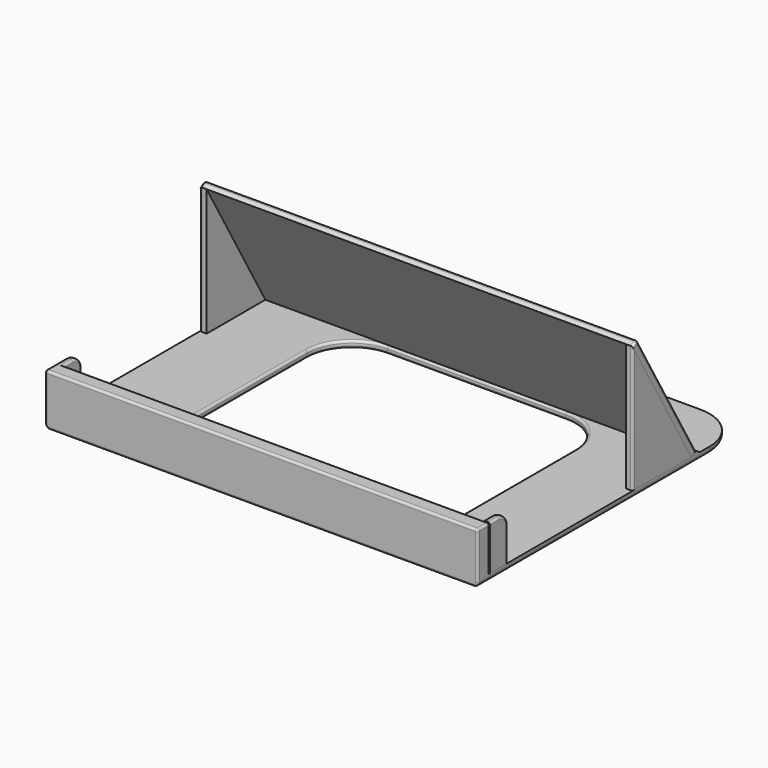
from build123d import *

# Parameters (mm, degrees)
F0_W          = 194
F0_H          = 150
F1_DEPTH      = 3
F2_W          = 6.9154556079
F2_H          = 20
F3_DEPTH      = 194
F5_DEPTH      = 3
F7_DEPTH      = 3
F8_W          = 194
F8_H          = 65.8179306876
F9_DEPTH      = 3
F11_DEPTH     = 194
F12_W         = 10
F12_H         = 20
F13_DEPTH     = 3
F14_R         = 5
F15_R         = 1
F16_R         = 1
F18_DEPTH     = 3
F19_R         = 1
F20_R         = 1
F21_R         = 1
F22_W         = 120
F22_H         = 112
F23_DEPTH     = 3.001
F24_R         = 20
F25_R         = 20
F26_R         = 2
F27_R         = 1
F28_R         = 1
F29_R         = 1
F30_T1_DEPTH  = 72
F30_T3_DEPTH  = 80
F30_T6_ANGLE  = 90
F30_T8_ANGLE  = 90
F30_T12_ANGLE = 111.4945483856
F30_T17_ANGLE = 111.4945483856
F31_R         = 1
F31_2_R       = 1


# Not quite as in the source:
# - a fillet or chamfer that OpenCascade refuses, or shapes differently, is made with other operations: its cross-section is extruded or revolved along the edge and cut away or added


with BuildPart() as f1:
    # F0 (on Top) → F1 (new body)
    with BuildSketch(Plane.XY):
        with Locations((8.0765881836, -7.0053721947)):
            Rectangle(F0_W, F0_H)
    extrude(amount=F1_DEPTH)

    # F2 (on face) → F3 (join)
    with BuildSketch(Plane(origin=(-88.9234118164, 0, 0), x_dir=(0, -1, 0), z_dir=(-1, 0, 0))):
        with Locations((78.5476443908, 13)):
            Rectangle(F2_W, F2_H)
    extrude(amount=-F3_DEPTH)

    # F4 (on face) → F5 (join)
    with BuildSketch(Plane(origin=(-88.9234118164, 0, 0), x_dir=(0, -1, 0), z_dir=(-1, 0, 0))):
        Polygon((-4.9100834131, 60), (-37.8190487569, 3), (-4.9100834131, 3), align=None)
    extrude(amount=-F5_DEPTH)

    # F12 (on face) → F13 (join)
    with BuildSketch(Plane(origin=(-88.9234118164, 0, 0), x_dir=(0, -1, 0), z_dir=(-1, 0, 0))):
        with Locations((70.0899165869, 13)):
            Rectangle(F12_W, F12_H)
    extrude(amount=-F13_DEPTH)

    # F14
    f14_edges = [f1.edges().sort_by_distance(p)[0] for p in [
        (-87.423412, -65.089917, 23),
    ]]
    fillet(f14_edges, radius=F14_R)

    # F21
    f21_edges = [f1.edges().sort_by_distance(p)[0] for p in [
        (8.076588, -82.005372, 23),
    ]]
    fillet(f21_edges, radius=F21_R)

    # F22 (on face) → F23 (cut, through all)
    with BuildSketch(Plane.XY.offset(3)):
        with Locations((9.5765881836, -19.0899165869)):
            Rectangle(F22_W, F22_H)
    extrude(amount=-F23_DEPTH, mode=Mode.SUBTRACT)

    # F24
    f24_edges = [f1.edges().sort_by_distance(p)[0] for p in [
        (-88.923412, 67.994628, 1.5),
        (105.076588, 67.994628, 1.5),
        (69.576588, 36.910083, 1.5),
        (-50.423412, 36.910083, 1.5),
    ]]
    fillet(f24_edges, radius=F24_R)

    # F25
    f25_edges = [f1.edges().sort_by_distance(p)[0] for p in [
        (69.576588, -75.089917, 1.5),
        (-50.423412, -75.089917, 1.5),
    ]]
    fillet(f25_edges, radius=F25_R)

    # F26
    f26_edges = [f1.edges().sort_by_distance(p)[0] for p in [
        (-88.923412, -17.005372, 0),
        (105.076588, -17.005372, 0),
        (99.218724, 62.136763, 0),
        (8.076588, 67.994628, 0),
        (-83.065547, 62.136763, 0),
    ]]
    fillet(f26_edges, radius=F26_R)

    # F27
    f27_edges = [f1.edges().sort_by_distance(p)[0] for p in [
        (-88.923412, 4.910083, 31.5),
    ]]
    fillet(f27_edges, radius=F27_R)

    # F28
    f28_edges = [f1.edges().sort_by_distance(p)[0] for p in [
        (-88.923412, -82.005372, 12),
        (-88.337625, -82.005372, 0.585786),
        (8.076588, -82.005372, 22),
        (8.076588, -82.005372, 0),
        (105.076588, -82.005372, 12),
        (104.490802, -82.005372, 0.585786),
    ]]
    fillet(f28_edges, radius=F28_R)

    # F29
    f29_edges = [f1.edges().sort_by_distance(p)[0] for p in [
        (-44.565547, -69.232052, 0),
        (63.718724, -69.232052, 0),
        (9.576588, -75.089917, 0),
        (63.718724, 31.052219, 0),
        (69.576588, -19.089917, 0),
        (9.576588, 36.910083, 0),
        (-44.565547, 31.052219, 0),
        (-50.423412, -19.089917, 0),
    ]]
    fillet(f29_edges, radius=F29_R)

    # F30: fillet of radius 1 on 6 edges, made by hand

    # F30_s2 → F30_t1 (cut)
    with BuildSketch(Plane.XZ.offset(-16.9100834131)):
        with BuildLine():
            ThreePointArc((-50.4234118164, 2), (-50.7163050352, 2.7071067812), (-51.4234118164, 3))
            Line((-51.4234118164, 3), (-50.4234118164, 3))
            Line((-50.4234118164, 3), (-50.4234118164, 2))
        make_face()
        with BuildLine():
            ThreePointArc((69.5765881836, 2), (69.8694814025, 2.7071067812), (70.5765881836, 3))
            Line((70.5765881836, 3), (69.5765881836, 3))
            Line((69.5765881836, 3), (69.5765881836, 2))
        make_face()
    extrude(amount=F30_T1_DEPTH, mode=Mode.SUBTRACT)

    # F30_s4 → F30_t3 (cut)
    with BuildSketch(Plane.YZ.offset(-30.4234118164)):
        with BuildLine():
            ThreePointArc((36.9100834131, 2), (37.2029766319, 2.7071067812), (37.9100834131, 3))
            Line((37.9100834131, 3), (36.9100834131, 3))
            Line((36.9100834131, 3), (36.9100834131, 2))
        make_face()
    extrude(amount=F30_T3_DEPTH, mode=Mode.SUBTRACT)

    # F30_s5 → F30_t6 (revolve, cut)
    with BuildSketch(Plane.YZ.offset(-30.4234118164)):
        with BuildLine():
            ThreePointArc((36.9100834131, 2), (37.2029766319, 2.7071067812), (37.9100834131, 3))
            Line((37.9100834131, 3), (36.9100834131, 3))
            Line((36.9100834131, 3), (36.9100834131, 2))
        make_face()
    revolve(axis=Axis((-30.4234118164, 16.9100834131, 3), (0, 0, 1)), revolution_arc=F30_T6_ANGLE, mode=Mode.SUBTRACT)

    # F30_s7 → F30_t8 (revolve, cut)
    with BuildSketch(Plane.XZ.offset(-16.9100834131)):
        with BuildLine():
            ThreePointArc((69.5765881836, 2), (69.8694814025, 2.7071067812), (70.5765881836, 3))
            Line((70.5765881836, 3), (69.5765881836, 3))
            Line((69.5765881836, 3), (69.5765881836, 2))
        make_face()
    revolve(axis=Axis((49.5765881836, 16.9100834131, 3), (0, 0, 1)), revolution_arc=F30_T8_ANGLE, mode=Mode.SUBTRACT)


with BuildPart() as f7:
    # F6 (on face) → F7 (new body)
    with BuildSketch(Plane.YZ.offset(105.0765881836)):
        Polygon((4.9100834131, 3), (37.8190487569, 3), (4.9100834131, 60), align=None)
    extrude(amount=-F7_DEPTH)

    # F20
    f20_edges = [f7.edges().sort_by_distance(p)[0] for p in [
        (105.076588, 4.910083, 31.5),
    ]]
    fillet(f20_edges, radius=F20_R)


with BuildPart() as f9:
    # F8 (on face) → F9 (new body)
    with BuildSketch(Plane(origin=(0, 29.6633246734, 17.1261284852), x_dir=(-1, 0, 0), z_dir=(0, 0.8660254038, 0.5))):
        with Locations((-8.0765881836, 16.5975171767)):
            Rectangle(F8_W, F8_H)
    extrude(amount=F9_DEPTH)

    # F15
    f15_edges = [f9.edges().sort_by_distance(p)[0] for p in [
        (8.076588, 7.50816, 61.5),
    ]]
    fillet(f15_edges, radius=F15_R)

    # F16
    f16_edges = [f9.edges().sort_by_distance(p)[0] for p in [
        (-88.923412, 24.212642, 32.566987),
    ]]
    fillet(f16_edges, radius=F16_R)

    # F19
    f19_edges = [f9.edges().sort_by_distance(p)[0] for p in [
        (105.076588, 24.212642, 32.566987),
    ]]
    fillet(f19_edges, radius=F19_R)


with BuildPart() as f11:
    # F10 (on face) → F11 (new body)
    with BuildSketch(Plane(origin=(-88.9234118164, 0, 0), x_dir=(0, -1, 0), z_dir=(-1, 0, 0))):
        Polygon((-37.8190487569, 3), (-40.4171249683, 4.5), (-42.5518223643, 3), align=None)
    extrude(amount=-F11_DEPTH)


with BuildPart() as f18:
    # F17 (on face) → F18 (new body)
    with BuildSketch(Plane.YZ.offset(105.0765881836)):
        with BuildLine():
            Line((-65.0899165869, 3), (-65.0899165869, 18))
            ThreePointArc((-65.0899165869, 18), (-66.5543826809, 21.5355339059), (-70.0899165869, 23))
            Line((-70.0899165869, 23), (-75.0899165869, 23))
            Line((-75.0899165869, 23), (-75.0899165869, 3))
            Line((-75.0899165869, 3), (-65.0899165869, 3))
        make_face()
    extrude(amount=-F18_DEPTH)

    # F31#2
    f31_2_edges = [f18.edges().sort_by_distance(p)[0] for p in [
        (105.076588, -65.089917, 10.5),
        (105.076588, -66.554383, 21.535534),
        (102.076588, -65.089917, 10.5),
        (102.076588, -66.554383, 21.535534),
        (105.076588, -72.589917, 23),
        (102.076588, -72.589917, 23),
    ]]
    fillet(f31_2_edges, radius=F31_2_R)


with BuildPart() as f30_tool10:
    # F30_s11 → F30_t12 (revolve)
    with BuildSketch(Plane.XZ.offset(55.0899165869)):
        with BuildLine():
            ThreePointArc((69.5765881836, 2), (69.8694814025, 2.7071067812), (70.5765881836, 3))
            Line((70.5765881836, 3), (69.5765881836, 3))
            Line((69.5765881836, 3), (69.5765881836, 2))
        make_face()
    revolve(axis=Axis((49.5765881836, -55.0899165869, 3), (0, 0, -1)), revolution_arc=F30_T12_ANGLE)

    split(bisect_by=Plane.XZ.offset(75.0899165869), keep=Keep.BOTTOM)


with BuildPart() as f1_1:
    add(f1.part)

    # F30_t9: cut F30_tool10
    add(f30_tool10.part, mode=Mode.SUBTRACT)


with BuildPart() as f30_tool15:
    # F30_s16 → F30_t17 (revolve)
    with BuildSketch(Plane(origin=(-45.1205998281, -17.7685178107, 0), x_dir=(0, 0, 1), z_dir=(0.9304524359, 0.3664126971, 0))):
        with BuildLine():
            ThreePointArc((2, 60.1110227003), (2.7071067812, 60.4039159191), (3, 61.1110227003))
            Line((3, 61.1110227003), (3, 60.1110227003))
            Line((3, 60.1110227003), (2, 60.1110227003))
        make_face()
    revolve(axis=Axis((-30.4234118164, -55.0899165869, 3), (0, 0, -1)), revolution_arc=F30_T17_ANGLE)

    split(bisect_by=Plane.XZ.offset(75.0899165869), keep=Keep.BOTTOM)


with BuildPart() as f1_2:
    add(f1_1.part)

    # F30_t14: cut F30_tool15
    add(f30_tool15.part, mode=Mode.SUBTRACT)

    # F31
    f31_edges = [f1_2.edges().sort_by_distance(p)[0] for p in [
        (-85.923412, -65.089917, 10.5),
        (9.076588, -75.089917, 23),
        (-85.923412, -72.589917, 23),
        (-85.923412, -66.554383, 21.535534),
    ]]
    fillet(f31_edges, radius=F31_R)


solid = Compound([f7.part, f9.part, f11.part, f18.part, f1_2.part])
